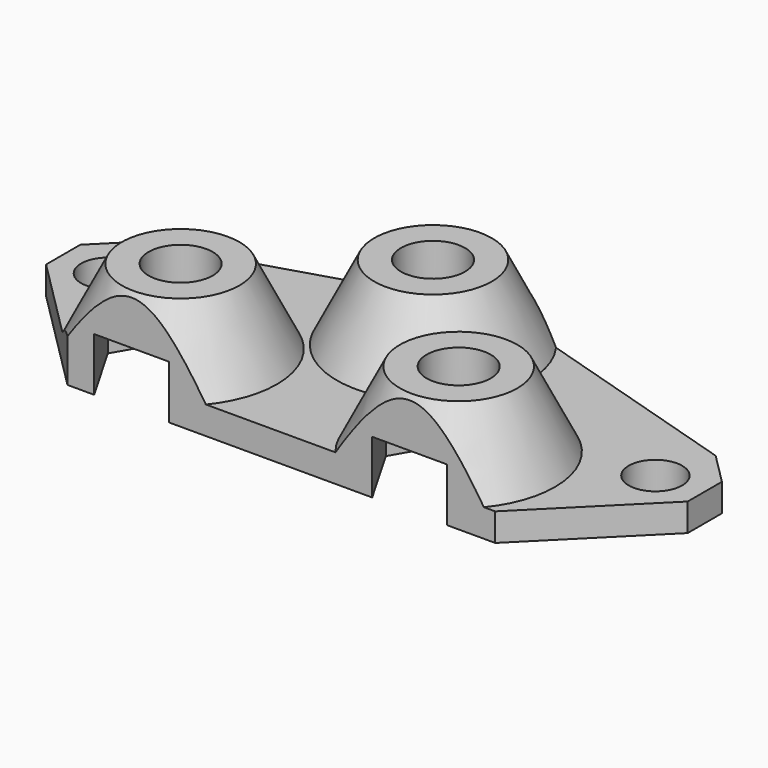
from build123d import *

# Parameters (mm, degrees)
F0_W     = 30
F0_H     = 12
F0_R     = 1.25
F1_DEPTH = 4.8
F2_R     = 1.5
F4_DEPTH = 4.8
F2_W     = 30
F2_H     = 12
F2_R_2   = 2.5
F2_R_3   = 1.25
F5_DEPTH = 3.5
F7_DEPTH = 2.5
F8_SIZE  = 5
F9_SIZE2 = 5
F9_SIZE  = 8


# Not quite as in the source:
# - a fillet or chamfer that OpenCascade refuses, or shapes differently, is made with other operations: its cross-section is extruded or revolved along the edge and cut away or added


with BuildPart() as f1:
    # F0 (on Top) → F1 (new body)
    with BuildSketch(Plane.XY):
        with Locations((0, 0.1359842196)):
            Rectangle(F0_W, F0_H)
        with Locations((-12.8, 0)):
            Circle(F0_R, mode=Mode.SUBTRACT)
        with Locations((12.8, 0)):
            Circle(F0_R, mode=Mode.SUBTRACT)
    extrude(amount=F1_DEPTH)

    # F2 (on face) → F4 (cut, through all)
    with BuildSketch(Plane.XY.offset(4.8)):
        with Locations((-7, -3)):
            Circle(F2_R)
        with Locations((0, 3)):
            Circle(F2_R)
        with Locations((6, -3)):
            Circle(F2_R)
    extrude(amount=-F4_DEPTH, mode=Mode.SUBTRACT)

    # F2 (on face) → F5 (cut)
    with BuildSketch(Plane.XY.offset(4.8)):
        with Locations((0, 0.1359842196)):
            Rectangle(F2_W, F2_H)
        with Locations((-7, -3)):
            Circle(F2_R_2, mode=Mode.SUBTRACT)
        with Locations((-12.8, 0)):
            Circle(F2_R_3, mode=Mode.SUBTRACT)
        with Locations((6, -3)):
            Circle(F2_R_2, mode=Mode.SUBTRACT)
        with Locations((12.8, 0)):
            Circle(F2_R_3, mode=Mode.SUBTRACT)
        with Locations((0, 3)):
            Circle(F2_R_2, mode=Mode.SUBTRACT)
    extrude(amount=-F5_DEPTH, mode=Mode.SUBTRACT)

    # F6: chamfer of 4 x 2 on 3 edges, made by hand


with BuildPart() as f6_tool2:
    # F6_s3 → F6_t4 (revolve)
    with BuildSketch(Plane.XZ.offset(3)):
        Polygon((-2.5, 1.3), (-4.5, 5.3), (-4.5, 1.3), align=None)
    revolve(axis=Axis((-7, -3, 1.3), (0, 0, 1)))

    split(bisect_by=Plane.XZ.offset(5.8640157804), keep=Keep.BOTTOM)

    split(bisect_by=Plane.XY.offset(4.8), keep=Keep.BOTTOM)


with BuildPart() as f1_1:
    add(f1.part)

    # F6_t1: union F6_tool2
    add(f6_tool2.part)


with BuildPart() as f6_tool8:
    # F6_s9 → F6_t10 (revolve)
    with BuildSketch(Plane.XZ.offset(-3)):
        Polygon((4.5, 1.3), (2.5, 5.3), (2.5, 1.3), align=None)
    revolve(axis=Axis((0, 3, 1.3), (0, 0, 1)))

    split(bisect_by=Plane.XZ.offset(-6.1359842196), keep=Keep.TOP)

    split(bisect_by=Plane.XY.offset(4.8), keep=Keep.BOTTOM)


with BuildPart() as f1_2:
    add(f1_1.part)

    # F6_t7: union F6_tool8
    add(f6_tool8.part)


with BuildPart() as f6_tool14:
    # F6_s15 → F6_t16 (revolve)
    with BuildSketch(Plane.XZ.offset(3)):
        Polygon((10.5, 1.3), (8.5, 5.3), (8.5, 1.3), align=None)
    revolve(axis=Axis((6, -3, 1.3), (0, 0, 1)))

    split(bisect_by=Plane.XZ.offset(5.8640157804), keep=Keep.BOTTOM)

    split(bisect_by=Plane.XY.offset(4.8), keep=Keep.BOTTOM)


with BuildPart() as f1_3:
    add(f1_2.part)

    # F6_t13: union F6_tool14
    add(f6_tool14.part)

    # F3 (on face) → F7 (cut)
    with BuildSketch(Plane(origin=(0, 0, 0), x_dir=(1, 0, 0), z_dir=(0, 0, -1))):
        Polygon((-5.2968167059, 5.95), (-8.7031832941, 5.95), (-8.7528263064, 5.8640157804), (-5.2471736936, 5.8640157804), align=None)
        Polygon((7.7528263064, 5.8640157804), (4.2471736936, 5.8640157804), (2.5936334118, 3), (4.2968167059, 0.05), (7.7031832941, 0.05), (9.4063665882, 3), align=None)
        Polygon((-1.7031832941, -5.95), (1.7031832941, -5.95), (3.4063665882, -3), (1.7031832941, -0.05), (-1.7031832941, -0.05), (-3.4063665882, -3), align=None)
        Polygon((-5.2471736936, 5.8640157804), (-8.7528263064, 5.8640157804), (-10.4063665882, 3), (-8.7031832941, 0.05), (-5.2968167059, 0.05), (-3.5936334118, 3), align=None)
    extrude(amount=-F7_DEPTH, mode=Mode.SUBTRACT)

    # F8 (call 1 of 4: OpenCascade refuses the feature's edges together)
    f8_edges = [f1_3.edges().sort_by_distance(p)[0] for p in [
        (-15, 6.135984, 0.65),
    ]]
    chamfer(f8_edges, length=F8_SIZE)

    # F8#2 (call 2 of 4)
    f8_2_edges = [f1_3.edges().sort_by_distance(p)[0] for p in [
        (-15, -5.864016, 0.65),
    ]]
    chamfer(f8_2_edges, length=F8_SIZE)

    # F8#3 (call 3 of 4)
    f8_3_edges = [f1_3.edges().sort_by_distance(p)[0] for p in [
        (15, 6.135984, 0.65),
    ]]
    chamfer(f8_3_edges, length=F8_SIZE)

    # F8#4 (call 4 of 4)
    f8_4_edges = [f1_3.edges().sort_by_distance(p)[0] for p in [
        (15, -5.864016, 0.65),
    ]]
    chamfer(f8_4_edges, length=F8_SIZE)

    # F9
    f9_edges = [f1_3.edges().sort_by_distance(p)[0] for p in [
        (10, 6.135984, 0.65),
        (-10, 6.135984, 0.65),
    ]]
    f9_side = f1_3.faces().sort_by_distance((0, 6.135984, 1.172283))[0]
    chamfer(f9_edges, length=F9_SIZE, length2=F9_SIZE2, reference=f9_side)


solid = f1_3.part
